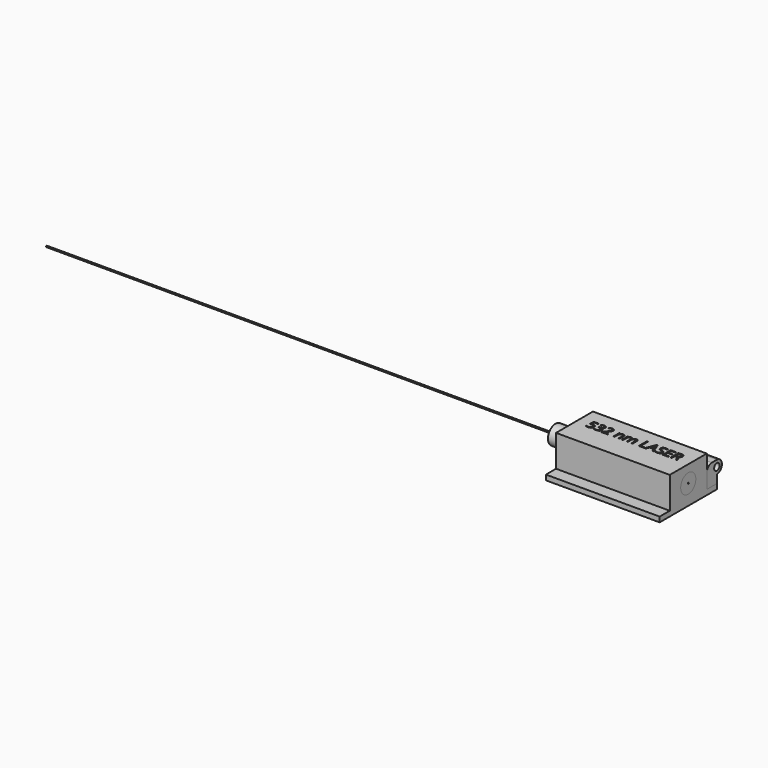
from build123d import *

# Parameters (mm, degrees)
F0_W      = 114.3
F0_H      = 12.7
F1_DEPTH  = 3.81
F3_DEPTH  = 4.572
F4_W      = 114.3
F4_H      = 6.35
F5_DEPTH  = 1.016
F7_DEPTH  = 11.684
F8_R      = 6.34999
F9_R      = 3.429
F9_R_2    = 9.525
F10_DEPTH = 114.301
F2_R      = 3.0988
F11_DEPTH = 10.668
F12_DEPTH = 114.3
F9_R_3    = 0.635
F13_DEPTH = 19.05
F15_DEPTH = 3.175
F16_DEPTH = 114.3
F17_DEPTH = 530.352


# Not quite as in the source:
# - a fillet or chamfer is up to 0.001 mm smaller than in the source, because OpenCascade refuses the exact size


with BuildPart() as f1:
    # F0 (on Top) → F1 (new body)
    with BuildSketch(Plane.XY):
        Rectangle(F0_W, F0_H)
    extrude(amount=F1_DEPTH)

    # F2 (on face) → F3 (join)
    with BuildSketch(Plane.XY.offset(3.81)):
        Polygon((-40.64, 6.2992), (-35.1847327765, 3.1496), (-35.1847327765, -3.1496), (-35.1847327765, -6.35), (35.1847327765, -6.35), (35.1847327765, -3.1496), (35.1847327765, 3.1496), (40.64, 6.2992), (46.0952672235, 3.1496), (46.0952672235, -3.1496), (46.0952672235, -6.35), (57.15, -6.35), (57.15, 6.35), (-57.15, 6.35), (-57.15, -6.35), (-46.0952672235, -6.35), (-46.0952672235, -3.1496), (-46.0952672235, 3.1496), align=None)
    extrude(amount=F3_DEPTH)

    # F4 (on face) → F5 (join)
    with BuildSketch(Plane.XY.offset(8.382)):
        with Locations((0, 9.525)):
            Rectangle(F4_W, F4_H)
        Polygon((-57.15, 6.35), (-57.15, -6.35), (-46.0952672235, -6.35), (-46.0952672235, 3.1496), (-40.64, 6.2992), (-35.1847327765, 3.1496), (-35.1847327765, -6.35), (35.1847327765, -6.35), (35.1847327765, 3.1496), (40.64, 6.2992), (46.0952672235, 3.1496), (46.0952672235, -6.35), (57.15, -6.35), (57.15, 6.35), align=None)
    extrude(amount=F5_DEPTH)

    # F6 (on face) → F7 (join)
    with BuildSketch(Plane.XY.offset(9.398)):
        Polygon((57.15, 12.7), (-57.15, 12.7), (-57.15, -6.35), (-46.0952672235, -6.35), (-46.0952672235, 3.1496), (-40.64, 6.2992), (-35.1847327765, 3.1496), (-35.1847327765, -6.35), (35.1847327765, -6.35), (35.1847327765, 3.1496), (40.64, 6.2992), (46.0952672235, 3.1496), (46.0952672235, -6.35), (57.15, -6.35), align=None)
        Polygon((35.1847327765, -6.35), (46.0952672235, -6.35), (46.0952672235, 3.1496), (40.64, 6.2992), (35.1847327765, 3.1496), align=None)
        Polygon((-46.0952672235, 3.1496), (-46.0952672235, -6.35), (-35.1847327765, -6.35), (-35.1847327765, 3.1496), (-40.64, 6.2992), align=None)
    extrude(amount=F7_DEPTH)

    # F8 (radius 6.35 in the source; OpenCascade refuses exactly that, so slightly less here)
    f8_edges = [f1.edges().sort_by_distance(p)[0] for p in [
        (0, 12.7, 21.082),
        (0, -6.35, 21.082),
        (0, 12.7, 8.382),
    ]]
    fillet(f8_edges, radius=F8_R)

    # F9 (on face) → F10 (cut, through all)
    with BuildSketch(Plane(origin=(-57.15, 0, 0), x_dir=(0, -1, 0), z_dir=(-1, 0, 0))):
        with Locations((-6.35, 14.732)):
            Circle(F9_R)
        Polygon((6.35, 0), (-6.35, 0), (-6.35, -5.1199872978), (65.491868, -5.1199872978), (65.491868, 0), (52.791868, 0), (52.791868, 31.7232050002), (6.35, 31.7232050002), align=None)
        with Locations((29.570934, 14.732)):
            Circle(F9_R_2, mode=Mode.SUBTRACT)
    extrude(amount=-F10_DEPTH, mode=Mode.SUBTRACT)

    # F2 (on face) → F11 (cut, symmetric)
    with BuildSketch(Plane.XY.offset(3.81)):
        with Locations((-40.64, 0)):
            Circle(F2_R)
        with Locations((40.64, 0)):
            Circle(F2_R)
    extrude(amount=F11_DEPTH, both=True, mode=Mode.SUBTRACT)


with BuildPart() as f12:
    # F9 (on face) → F12 (new body)
    with BuildSketch(Plane(origin=(-57.15, 0, 0), x_dir=(0, -1, 0), z_dir=(-1, 0, 0))):
        Polygon((6.35, 0), (-6.35, 0), (-6.35, -5.1199872978), (65.491868, -5.1199872978), (65.491868, 0), (52.791868, 0), (52.791868, 31.7232050002), (6.35, 31.7232050002), (6.35, 14.73201), align=None)
        with Locations((29.570934, 14.732)):
            Circle(F9_R_2, mode=Mode.SUBTRACT)
    extrude(amount=-F12_DEPTH)

    # F9 (on face) → F13 (join, symmetric)
    with BuildSketch(Plane(origin=(-57.15, 0, 0), x_dir=(0, -1, 0), z_dir=(-1, 0, 0))):
        with Locations((29.570934, 14.732)):
            Circle(F9_R_2)
        with Locations((29.570934, 14.732)):
            Circle(F9_R_3, mode=Mode.SUBTRACT)
    extrude(amount=F13_DEPTH, both=True)

    # F14 (on face) → F15 (cut)
    with BuildSketch(Plane.XY.offset(31.7232050002)):
        with BuildLine():
            Line((-45.282163951, -29.570934), (-42.5031012768, -29.570934))
            add(Edge.make_bspline(
                [(-41.0225434028, -28.8201787917), (-41.624680638, -29.3583014371), (-42.5031012768, -29.570934)],
                knots=[0, 0, 0, 0.6048622658, 0.6048622658, 0.6048622658], degree=2))
            add(Edge.make_bspline(
                [(-40.0270486111, -26.3672708056), (-40.0270486111, -27.9305173333), (-41.0225434028, -28.8201787917)],
                knots=[0, 0, 0, 1, 1, 1], degree=2))
            add(Edge.make_bspline(
                [(-40.9398611111, -24.2065069167), (-40.0270486111, -24.9958471944), (-40.0270486111, -26.3672708056)],
                knots=[0, 0, 0, 1, 1, 1], degree=2))
            add(Edge.make_bspline(
                [(-43.4445833333, -23.4171666389), (-41.8526736111, -23.4171666389), (-40.9398611111, -24.2065069167)],
                knots=[0, 0, 0, 1, 1, 1], degree=2))
            add(Edge.make_bspline(
                [(-45.0232638889, -23.5759166389), (-44.23171875, -23.4171666389), (-43.4445833333, -23.4171666389)],
                knots=[0, 0, 0, 1, 1, 1], degree=2))
            Line((-45.0232638889, -23.5759166389), (-44.7675, -20.5508471944))
            Line((-44.7675, -20.5508471944), (-40.7370138889, -20.5508471944))
            Line((-40.7370138889, -20.5508471944), (-40.7370138889, -19.4969235833))
            Line((-40.7370138889, -19.4969235833), (-45.7464583333, -19.4969235833))
            Line((-45.7464583333, -19.4969235833), (-46.1256944444, -24.2109166389))
            Line((-46.1256944444, -24.2109166389), (-45.5325868056, -24.59015275))
            add(Edge.make_bspline(
                [(-43.7819270833, -24.3895103889), (-44.4367708333, -24.3895103889), (-45.5325868056, -24.59015275)],
                knots=[0, 0, 0, 1, 1, 1], degree=2))
            add(Edge.make_bspline(
                [(-41.2000347222, -26.4973576111), (-41.2000347222, -24.3895103889), (-43.7819270833, -24.3895103889)],
                knots=[0, 0, 0, 1, 1, 1], degree=2))
            add(Edge.make_bspline(
                [(-41.8714149306, -28.152105875), (-41.2000347222, -27.5799444167), (-41.2000347222, -26.4973576111)],
                knots=[0, 0, 0, 1, 1, 1], degree=2))
            add(Edge.make_bspline(
                [(-43.75546875, -28.7242673333), (-42.5427951389, -28.7242673333), (-41.8714149306, -28.152105875)],
                knots=[0, 0, 0, 1, 1, 1], degree=2))
            add(Edge.make_bspline(
                [(-45.1687847222, -28.5478784444), (-44.4522048611, -28.7242673333), (-43.75546875, -28.7242673333)],
                knots=[0, 0, 0, 1, 1, 1], degree=2))
            add(Edge.make_bspline(
                [(-46.3660243056, -28.062809), (-45.8853645833, -28.3714895556), (-45.1687847222, -28.5478784444)],
                knots=[0, 0, 0, 1, 1, 1], degree=2))
            Line((-46.3660243056, -28.062809), (-46.3660243056, -29.1652395556))
            add(Edge.make_bspline(
                [(-45.282163951, -29.570934), (-45.9229450337, -29.4347976347), (-46.3660243056, -29.1652395556)],
                knots=[0.5050353738, 0.5050353738, 0.5050353738, 1, 1, 1], degree=2))
        make_face()
        with BuildLine():
            Line((-37.3682522224, -29.570934), (-34.4058239367, -29.570934))
            add(Edge.make_bspline(
                [(-32.9736979167, -28.9337291389), (-33.549949731, -29.3815009681), (-34.4058239367, -29.570934)],
                knots=[0, 0, 0, 0.5769429439, 0.5769429439, 0.5769429439], degree=2))
            add(Edge.make_bspline(
                [(-31.9748958333, -26.7178437222), (-31.9748958333, -28.1576180278), (-32.9736979167, -28.9337291389)],
                knots=[0, 0, 0, 1, 1, 1], degree=2))
            add(Edge.make_bspline(
                [(-32.5602864583, -25.0917586528), (-31.9748958333, -25.7124270556), (-31.9748958333, -26.7178437222)],
                knots=[0, 0, 0, 1, 1, 1], degree=2))
            add(Edge.make_bspline(
                [(-34.3583506944, -24.3211596944), (-33.1456770833, -24.47109025), (-32.5602864583, -25.0917586528)],
                knots=[0, 0, 0, 1, 1, 1], degree=2))
            Line((-34.3583506944, -24.3211596944), (-34.3583506944, -24.2660381667))
            add(Edge.make_bspline(
                [(-32.8248697917, -23.4458298333), (-33.3661631944, -24.0587812222), (-34.3583506944, -24.2660381667)],
                knots=[0, 0, 0, 1, 1, 1], degree=2))
            add(Edge.make_bspline(
                [(-32.2835763889, -21.8671492778), (-32.2835763889, -22.8328784444), (-32.8248697917, -23.4458298333)],
                knots=[0, 0, 0, 1, 1, 1], degree=2))
            add(Edge.make_bspline(
                [(-33.0971701389, -20.0249878194), (-32.2835763889, -20.6963680278), (-32.2835763889, -21.8671492778)],
                knots=[0, 0, 0, 1, 1, 1], degree=2))
            add(Edge.make_bspline(
                [(-35.3769965278, -19.3536076111), (-33.9107638889, -19.3536076111), (-33.0971701389, -20.0249878194)],
                knots=[0, 0, 0, 1, 1, 1], degree=2))
            add(Edge.make_bspline(
                [(-37.0835590278, -19.6325225417), (-36.274375, -19.3536076111), (-35.3769965278, -19.3536076111)],
                knots=[0, 0, 0, 1, 1, 1], degree=2))
            add(Edge.make_bspline(
                [(-38.5123090278, -20.4009166389), (-37.8927430556, -19.9114374722), (-37.0835590278, -19.6325225417)],
                knots=[0, 0, 0, 1, 1, 1], degree=2))
            Line((-38.5123090278, -20.4009166389), (-37.9346354167, -21.1726180278))
            add(Edge.make_bspline(
                [(-36.5973871528, -20.5100572639), (-37.1827777778, -20.6897534444), (-37.9346354167, -21.1726180278)],
                knots=[0, 0, 0, 1, 1, 1], degree=2))
            add(Edge.make_bspline(
                [(-35.3505381944, -20.3303610833), (-36.0119965278, -20.3303610833), (-36.5973871528, -20.5100572639)],
                knots=[0, 0, 0, 1, 1, 1], degree=2))
            add(Edge.make_bspline(
                [(-33.9758072917, -20.7514895556), (-34.4818229167, -20.3303610833), (-35.3505381944, -20.3303610833)],
                knots=[0, 0, 0, 1, 1, 1], degree=2))
            add(Edge.make_bspline(
                [(-33.4697916667, -21.9090416389), (-33.4697916667, -21.1726180278), (-33.9758072917, -20.7514895556)],
                knots=[0, 0, 0, 1, 1, 1], degree=2))
            add(Edge.make_bspline(
                [(-34.1588107639, -23.3532256667), (-33.4697916667, -22.8328784444), (-33.4697916667, -21.9090416389)],
                knots=[0, 0, 0, 1, 1, 1], degree=2))
            add(Edge.make_bspline(
                [(-36.0252256944, -23.8735728889), (-34.8478298611, -23.8735728889), (-34.1588107639, -23.3532256667)],
                knots=[0, 0, 0, 1, 1, 1], degree=2))
            Line((-36.0252256944, -23.8735728889), (-37.0306423611, -23.8735728889))
            Line((-37.0306423611, -23.8735728889), (-37.0306423611, -24.8569409444))
            Line((-37.0306423611, -24.8569409444), (-36.0384548611, -24.8569409444))
            add(Edge.make_bspline(
                [(-33.15890625, -26.6913853889), (-33.15890625, -24.8569409444), (-36.0384548611, -24.8569409444)],
                knots=[0, 0, 0, 1, 1, 1], degree=2))
            add(Edge.make_bspline(
                [(-35.7694618056, -28.7374965), (-33.15890625, -28.7374965), (-33.15890625, -26.6913853889)],
                knots=[0, 0, 0, 1, 1, 1], degree=2))
            add(Edge.make_bspline(
                [(-37.1717534722, -28.568824625), (-36.4309201389, -28.7374965), (-35.7694618056, -28.7374965)],
                knots=[0, 0, 0, 1, 1, 1], degree=2))
            add(Edge.make_bspline(
                [(-38.5674305556, -28.0760381667), (-37.9125868056, -28.40015275), (-37.1717534722, -28.568824625)],
                knots=[0, 0, 0, 1, 1, 1], degree=2))
            Line((-38.5674305556, -28.0760381667), (-38.5674305556, -29.1652395556))
            add(Edge.make_bspline(
                [(-37.3682522224, -29.570934), (-37.9845576037, -29.4464141838), (-38.5674305556, -29.1652395556)],
                knots=[0.0691615274, 0.0691615274, 0.0691615274, 1, 1, 1], degree=2))
        make_face()
        with BuildLine():
            Line((-30.4579513889, -28.5853610833), (-30.4579513889, -29.570934))
            Line((-30.4579513889, -29.570934), (-23.8367534722, -29.570934))
            Line((-23.8367534722, -29.570934), (-23.8367534722, -28.5103958056))
            Line((-23.8367534722, -28.5103958056), (-29.0181770833, -28.5103958056))
            Line((-29.0181770833, -28.5103958056), (-29.0181770833, -28.4552742778))
            Line((-29.0181770833, -28.4552742778), (-26.8133159722, -26.2989201111))
            add(Edge.make_bspline(
                [(-24.8024826389, -23.9286944167), (-25.34046875, -24.8657603889), (-26.8133159722, -26.2989201111)],
                knots=[0, 0, 0, 1, 1, 1], degree=2))
            add(Edge.make_bspline(
                [(-24.2644965278, -22.0325138611), (-24.2644965278, -22.9916284444), (-24.8024826389, -23.9286944167)],
                knots=[0, 0, 0, 1, 1, 1], degree=2))
            add(Edge.make_bspline(
                [(-25.0703732639, -20.0801093472), (-24.2644965278, -20.8066110833), (-24.2644965278, -22.0325138611)],
                knots=[0, 0, 0, 1, 1, 1], degree=2))
            add(Edge.make_bspline(
                [(-27.2961805556, -19.3536076111), (-25.87625, -19.3536076111), (-25.0703732639, -20.0801093472)],
                knots=[0, 0, 0, 1, 1, 1], degree=2))
            add(Edge.make_bspline(
                [(-30.3278645833, -20.5111596944), (-28.9365972222, -19.3536076111), (-27.2961805556, -19.3536076111)],
                knots=[0, 0, 0, 1, 1, 1], degree=2))
            Line((-30.3278645833, -20.5111596944), (-29.7215277778, -21.2894756667))
            add(Edge.make_bspline(
                [(-28.4713715278, -20.5376180278), (-29.0336111111, -20.7448749722), (-29.7215277778, -21.2894756667)],
                knots=[0, 0, 0, 1, 1, 1], degree=2))
            add(Edge.make_bspline(
                [(-27.2829513889, -20.3303610833), (-27.9091319444, -20.3303610833), (-28.4713715278, -20.5376180278)],
                knots=[0, 0, 0, 1, 1, 1], degree=2))
            add(Edge.make_bspline(
                [(-25.9247569444, -20.8022013611), (-26.4142361111, -20.3303610833), (-27.2829513889, -20.3303610833)],
                knots=[0, 0, 0, 1, 1, 1], degree=2))
            add(Edge.make_bspline(
                [(-25.4352777778, -22.0810208056), (-25.4352777778, -21.2740416389), (-25.9247569444, -20.8022013611)],
                knots=[0, 0, 0, 1, 1, 1], degree=2))
            add(Edge.make_bspline(
                [(-25.628203125, -23.1481735833), (-25.4352777778, -22.6520798333), (-25.4352777778, -22.0810208056)],
                knots=[0, 0, 0, 1, 1, 1], degree=2))
            add(Edge.make_bspline(
                [(-26.2069791667, -24.1679218472), (-25.8211284722, -23.6442673333), (-25.628203125, -23.1481735833)],
                knots=[0, 0, 0, 1, 1, 1], degree=2))
            add(Edge.make_bspline(
                [(-27.8055034722, -25.919684), (-26.5928298611, -24.6915763611), (-26.2069791667, -24.1679218472)],
                knots=[0, 0, 0, 1, 1, 1], degree=2))
            Line((-27.8055034722, -25.919684), (-30.4579513889, -28.5853610833))
        make_face()
        with BuildLine():
            Line((-18.2011284722, -22.0192846944), (-18.2011284722, -29.570934))
            Line((-18.2011284722, -29.570934), (-17.0568055556, -29.570934))
            Line((-17.0568055556, -29.570934), (-17.0568055556, -25.6087985833))
            add(Edge.make_bspline(
                [(-16.5055902778, -23.4932343472), (-17.0568055556, -24.1337465), (-17.0568055556, -25.6087985833)],
                knots=[0, 0, 0, 1, 1, 1], degree=2))
            add(Edge.make_bspline(
                [(-14.7703645833, -22.8527221944), (-15.954375, -22.8527221944), (-16.5055902778, -23.4932343472)],
                knots=[0, 0, 0, 1, 1, 1], degree=2))
            add(Edge.make_bspline(
                [(-13.4529600694, -23.3080260139), (-13.8729861111, -22.8527221944), (-14.7703645833, -22.8527221944)],
                knots=[0, 0, 0, 1, 1, 1], degree=2))
            add(Edge.make_bspline(
                [(-13.0329340278, -24.6849617778), (-13.0329340278, -23.7633298333), (-13.4529600694, -23.3080260139)],
                knots=[0, 0, 0, 1, 1, 1], degree=2))
            Line((-13.0329340278, -24.6849617778), (-13.0329340278, -29.570934))
            Line((-13.0329340278, -29.570934), (-11.8886111111, -29.570934))
            Line((-11.8886111111, -29.570934), (-11.8886111111, -24.6452742778))
            add(Edge.make_bspline(
                [(-12.5776302083, -22.5385294861), (-11.8886111111, -23.1966805278), (-11.8886111111, -24.6452742778)],
                knots=[0, 0, 0, 1, 1, 1], degree=2))
            add(Edge.make_bspline(
                [(-14.6314583333, -21.8803784444), (-13.2666493056, -21.8803784444), (-12.5776302083, -22.5385294861)],
                knots=[0, 0, 0, 1, 1, 1], degree=2))
            add(Edge.make_bspline(
                [(-16.043671875, -22.1879565694), (-15.4097743056, -21.8803784444), (-14.6314583333, -21.8803784444)],
                knots=[0, 0, 0, 1, 1, 1], degree=2))
            add(Edge.make_bspline(
                [(-17.0303472222, -23.0533645556), (-16.6775694444, -22.4955346944), (-16.043671875, -22.1879565694)],
                knots=[0, 0, 0, 1, 1, 1], degree=2))
            Line((-17.0303472222, -23.0533645556), (-17.08546875, -23.0533645556))
            Line((-17.08546875, -23.0533645556), (-17.2706770833, -22.0192846944))
            Line((-17.2706770833, -22.0192846944), (-18.2011284722, -22.0192846944))
        make_face()
        with BuildLine():
            Line((-9.5404340278, -22.0192846944), (-9.5404340278, -29.570934))
            Line((-9.5404340278, -29.570934), (-8.3961111111, -29.570934))
            Line((-8.3961111111, -29.570934), (-8.3961111111, -25.6087985833))
            add(Edge.make_bspline(
                [(-7.8967100694, -23.4965416389), (-8.3961111111, -24.1403610833), (-8.3961111111, -25.6087985833)],
                knots=[0, 0, 0, 1, 1, 1], degree=2))
            add(Edge.make_bspline(
                [(-6.3235416667, -22.8527221944), (-7.3973090278, -22.8527221944), (-7.8967100694, -23.4965416389)],
                knots=[0, 0, 0, 1, 1, 1], degree=2))
            add(Edge.make_bspline(
                [(-5.1174826389, -23.3036162917), (-5.5033333333, -22.8527221944), (-6.3235416667, -22.8527221944)],
                knots=[0, 0, 0, 1, 1, 1], degree=2))
            add(Edge.make_bspline(
                [(-4.7316319444, -24.6585034444), (-4.7316319444, -23.7545103889), (-5.1174826389, -23.3036162917)],
                knots=[0, 0, 0, 1, 1, 1], degree=2))
            Line((-4.7316319444, -24.6585034444), (-4.7316319444, -29.570934))
            Line((-4.7316319444, -29.570934), (-3.5873090278, -29.570934))
            Line((-3.5873090278, -29.570934), (-3.5873090278, -25.3530346944))
            add(Edge.make_bspline(
                [(-3.0768836806, -23.4656735833), (-3.5873090278, -24.0786249722), (-3.5873090278, -25.3530346944)],
                knots=[0, 0, 0, 1, 1, 1], degree=2))
            add(Edge.make_bspline(
                [(-1.4993055556, -22.8527221944), (-2.5664583333, -22.8527221944), (-3.0768836806, -23.4656735833)],
                knots=[0, 0, 0, 1, 1, 1], degree=2))
            add(Edge.make_bspline(
                [(-0.2998611111, -23.3036162917), (-0.6857118056, -22.8527221944), (-1.4993055556, -22.8527221944)],
                knots=[0, 0, 0, 1, 1, 1], degree=2))
            add(Edge.make_bspline(
                [(0.0859895833, -24.6585034444), (0.0859895833, -23.7545103889), (-0.2998611111, -23.3036162917)],
                knots=[0, 0, 0, 1, 1, 1], degree=2))
            Line((0.0859895833, -24.6585034444), (0.0859895833, -29.570934))
            Line((0.0859895833, -29.570934), (1.2281076389, -29.570934))
            Line((1.2281076389, -29.570934), (1.2281076389, -24.6452742778))
            add(Edge.make_bspline(
                [(0.5909027778, -22.5385294861), (1.2281076389, -23.1966805278), (1.2281076389, -24.6452742778)],
                knots=[0, 0, 0, 1, 1, 1], degree=2))
            add(Edge.make_bspline(
                [(-1.3273263889, -21.8803784444), (-0.0463020833, -21.8803784444), (0.5909027778, -22.5385294861)],
                knots=[0, 0, 0, 1, 1, 1], degree=2))
            add(Edge.make_bspline(
                [(-2.788046875, -22.2254392083), (-2.1475347222, -21.8803784444), (-1.3273263889, -21.8803784444)],
                knots=[0, 0, 0, 1, 1, 1], degree=2))
            add(Edge.make_bspline(
                [(-3.7659027778, -23.1636076111), (-3.4285590278, -22.5704999722), (-2.788046875, -22.2254392083)],
                knots=[0, 0, 0, 1, 1, 1], degree=2))
            Line((-3.7659027778, -23.1636076111), (-3.8210243056, -23.1636076111))
            add(Edge.make_bspline(
                [(-6.1361284722, -21.8803784444), (-4.365625, -21.8803784444), (-3.8210243056, -23.1636076111)],
                knots=[0, 0, 0, 1, 1, 1], degree=2))
            add(Edge.make_bspline(
                [(-7.4557378472, -22.1912638611), (-6.8659375, -21.8803784444), (-6.1361284722, -21.8803784444)],
                knots=[0, 0, 0, 1, 1, 1], degree=2))
            add(Edge.make_bspline(
                [(-8.3696527778, -23.0533645556), (-8.0455381944, -22.5021492778), (-7.4557378472, -22.1912638611)],
                knots=[0, 0, 0, 1, 1, 1], degree=2))
            Line((-8.3696527778, -23.0533645556), (-8.4247743056, -23.0533645556))
            Line((-8.4247743056, -23.0533645556), (-8.6099826389, -22.0192846944))
            Line((-8.6099826389, -22.0192846944), (-9.5404340278, -22.0192846944))
        make_face()
        Polygon((7.4237673611, -19.4969235833), (7.4237673611, -29.570934), (13.0395486111, -29.570934), (13.0395486111, -28.5103958056), (8.5945486111, -28.5103958056), (8.5945486111, -19.4969235833), align=None)
        Polygon((17.3456423611, -19.4550312222), (13.3636631944, -29.570934), (14.5498784722, -29.570934), (15.7890104167, -26.3672708056), (19.8261111111, -26.3672708056), (21.0806770833, -29.570934), (22.2933506944, -29.570934), (18.3312152778, -19.4550312222), align=None)
        with BuildLine():
            Line((18.2893229167, -22.1912638611), (19.4623090278, -25.3133471944))
            Line((19.4623090278, -25.3133471944), (16.2035243056, -25.3133471944))
            Line((16.2035243056, -25.3133471944), (17.3875347222, -22.1912638611))
            add(Edge.make_bspline(
                [(17.8218923611, -20.7382603889), (17.6697569444, -21.3997187222), (17.3875347222, -22.1912638611)],
                knots=[0, 0, 0, 1, 1, 1], degree=2))
            add(Edge.make_bspline(
                [(18.2893229167, -22.1912638611), (18.0622222222, -21.5981562222), (17.8218923611, -20.7382603889)],
                knots=[0, 0, 0, 1, 1, 1], degree=2))
        make_face(mode=Mode.SUBTRACT)
        with BuildLine():
            Line((24.065394409, -29.570934), (27.0786655087, -29.570934))
            add(Edge.make_bspline(
                [(28.3975086806, -28.9645971944), (27.8493399544, -29.3880966903), (27.0786655087, -29.570934)],
                knots=[0, 0, 0, 0.5682703015, 0.5682703015, 0.5682703015], degree=2))
            add(Edge.make_bspline(
                [(29.3621354167, -26.8898228889), (29.3621354167, -28.2193541389), (28.3975086806, -28.9645971944)],
                knots=[0, 0, 0, 1, 1, 1], degree=2))
            add(Edge.make_bspline(
                [(28.7668229167, -25.2097187222), (29.3621354167, -25.8579478889), (29.3621354167, -26.8898228889)],
                knots=[0, 0, 0, 1, 1, 1], degree=2))
            add(Edge.make_bspline(
                [(26.5862152778, -23.9970451111), (28.1715104167, -24.5614895556), (28.7668229167, -25.2097187222)],
                knots=[0, 0, 0, 1, 1, 1], degree=2))
            add(Edge.make_bspline(
                [(25.1839236111, -23.3807864306), (25.6425347222, -23.6597013611), (26.5862152778, -23.9970451111)],
                knots=[0, 0, 0, 1, 1, 1], degree=2))
            add(Edge.make_bspline(
                [(24.5323871528, -22.7667326111), (24.7253125, -23.1018715), (25.1839236111, -23.3807864306)],
                knots=[0, 0, 0, 1, 1, 1], degree=2))
            add(Edge.make_bspline(
                [(24.3394618056, -21.9090416389), (24.3394618056, -22.4315937222), (24.5323871528, -22.7667326111)],
                knots=[0, 0, 0, 1, 1, 1], degree=2))
            add(Edge.make_bspline(
                [(24.8631163194, -20.7999965), (24.3394618056, -21.1990763611), (24.3394618056, -21.9090416389)],
                knots=[0, 0, 0, 1, 1, 1], degree=2))
            add(Edge.make_bspline(
                [(26.3172222222, -20.4009166389), (25.3867708333, -20.4009166389), (24.8631163194, -20.7999965)],
                knots=[0, 0, 0, 1, 1, 1], degree=2))
            add(Edge.make_bspline(
                [(28.7425694444, -20.9234687222), (27.4946180556, -20.4009166389), (26.3172222222, -20.4009166389)],
                knots=[0, 0, 0, 1, 1, 1], degree=2))
            Line((28.7425694444, -20.9234687222), (29.1085763889, -19.9048228889))
            add(Edge.make_bspline(
                [(26.3458854167, -19.3536076111), (27.8473958333, -19.3536076111), (29.1085763889, -19.9048228889)],
                knots=[0, 0, 0, 1, 1, 1], degree=2))
            add(Edge.make_bspline(
                [(24.0296788194, -20.0426267083), (24.90390625, -19.3536076111), (26.3458854167, -19.3536076111)],
                knots=[0, 0, 0, 1, 1, 1], degree=2))
            add(Edge.make_bspline(
                [(23.1554513889, -21.8958124722), (23.1554513889, -20.7316458056), (24.0296788194, -20.0426267083)],
                knots=[0, 0, 0, 1, 1, 1], degree=2))
            add(Edge.make_bspline(
                [(23.7584809028, -23.6938767083), (23.1554513889, -23.0048576111), (23.1554513889, -21.8958124722)],
                knots=[0, 0, 0, 1, 1, 1], degree=2))
            add(Edge.make_bspline(
                [(25.7660069444, -24.8856041389), (24.3615104167, -24.3828958056), (23.7584809028, -23.6938767083)],
                knots=[0, 0, 0, 1, 1, 1], degree=2))
            add(Edge.make_bspline(
                [(27.2642100694, -25.5261162917), (26.7714236111, -25.2427916389), (25.7660069444, -24.8856041389)],
                knots=[0, 0, 0, 1, 1, 1], degree=2))
            add(Edge.make_bspline(
                [(27.9675607639, -26.1434774028), (27.7569965278, -25.8094409444), (27.2642100694, -25.5261162917)],
                knots=[0, 0, 0, 1, 1, 1], degree=2))
            add(Edge.make_bspline(
                [(28.178125, -27.0000659444), (28.178125, -26.4775138611), (27.9675607639, -26.1434774028)],
                knots=[0, 0, 0, 1, 1, 1], degree=2))
            add(Edge.make_bspline(
                [(27.5850173611, -28.2380954583), (28.178125, -27.7938159444), (28.178125, -27.0000659444)],
                knots=[0, 0, 0, 1, 1, 1], degree=2))
            add(Edge.make_bspline(
                [(25.8211284722, -28.6823749722), (26.9919097222, -28.6823749722), (27.5850173611, -28.2380954583)],
                knots=[0, 0, 0, 1, 1, 1], degree=2))
            add(Edge.make_bspline(
                [(24.3747395833, -28.5302395556), (25.1045486111, -28.6823749722), (25.8211284722, -28.6823749722)],
                knots=[0, 0, 0, 1, 1, 1], degree=2))
            add(Edge.make_bspline(
                [(23.0231597222, -28.1179305278), (23.6449305556, -28.3781041389), (24.3747395833, -28.5302395556)],
                knots=[0, 0, 0, 1, 1, 1], degree=2))
            Line((23.0231597222, -28.1179305278), (23.0231597222, -29.2468194167))
            add(Edge.make_bspline(
                [(24.065394409, -29.570934), (23.4599372399, -29.456233295), (23.0231597222, -29.2468194167)],
                knots=[0.5477225575, 0.5477225575, 0.5477225575, 1, 1, 1], degree=2))
        make_face()
        Polygon((31.4236805556, -29.570934), (37.0394618056, -29.570934), (37.0394618056, -28.5236249722), (32.5944618056, -28.5236249722), (32.5944618056, -24.8172534444), (36.77046875, -24.8172534444), (36.77046875, -23.7831735833), (32.5944618056, -23.7831735833), (32.5944618056, -20.5376180278), (37.0394618056, -20.5376180278), (37.0394618056, -19.4969235833), (31.4236805556, -19.4969235833), align=None)
        with BuildLine():
            Line((44.9835763889, -29.570934), (46.3682291667, -29.570934))
            Line((46.3682291667, -29.570934), (43.6319965278, -25.0443541389))
            add(Edge.make_bspline(
                [(45.6582638889, -22.3433992778), (45.6582638889, -24.3410034444), (43.6319965278, -25.0443541389)],
                knots=[0, 0, 0, 1, 1, 1], degree=2))
            add(Edge.make_bspline(
                [(44.7730121528, -20.2068888611), (45.6582638889, -20.9168541389), (45.6582638889, -22.3433992778)],
                knots=[0, 0, 0, 1, 1, 1], degree=2))
            add(Edge.make_bspline(
                [(42.0334722222, -19.4969235833), (43.8877604167, -19.4969235833), (44.7730121528, -20.2068888611)],
                knots=[0, 0, 0, 1, 1, 1], degree=2))
            Line((42.0334722222, -19.4969235833), (39.27078125, -19.4969235833))
            Line((39.27078125, -19.4969235833), (39.27078125, -29.570934))
            Line((39.27078125, -29.570934), (40.4415625, -29.570934))
            Line((40.4415625, -29.570934), (40.4415625, -25.3816978889))
            Line((40.4415625, -25.3816978889), (42.545, -25.3816978889))
            Line((42.545, -25.3816978889), (44.9835763889, -29.570934))
        make_face()
        with BuildLine():
            Line((42.04890625, -24.3762812222), (40.4415625, -24.3762812222))
            Line((40.4415625, -24.3762812222), (40.4415625, -20.5243888611))
            Line((40.4415625, -20.5243888611), (41.9651215278, -20.5243888611))
            add(Edge.make_bspline(
                [(43.8568923611, -20.9653610833), (43.2681944444, -20.5243888611), (41.9651215278, -20.5243888611)],
                knots=[0, 0, 0, 1, 1, 1], degree=2))
            add(Edge.make_bspline(
                [(44.4455902778, -22.4051353889), (44.4455902778, -21.4063333056), (43.8568923611, -20.9653610833)],
                knots=[0, 0, 0, 1, 1, 1], degree=2))
            add(Edge.make_bspline(
                [(43.8668142361, -23.8834947639), (44.4455902778, -23.3907083056), (44.4455902778, -22.4051353889)],
                knots=[0, 0, 0, 1, 1, 1], degree=2))
            add(Edge.make_bspline(
                [(42.04890625, -24.3762812222), (43.2880381944, -24.3762812222), (43.8668142361, -23.8834947639)],
                knots=[0, 0, 0, 1, 1, 1], degree=2))
        make_face(mode=Mode.SUBTRACT)
    extrude(amount=-F15_DEPTH, mode=Mode.SUBTRACT)

    # F9 (on face) → F16 (join)
    with BuildSketch(Plane(origin=(-57.15, 0, 0), x_dir=(0, -1, 0), z_dir=(-1, 0, 0))):
        with Locations((29.570934, 14.732)):
            Circle(F9_R_2)
        with Locations((29.570934, 14.732)):
            Circle(F9_R_3, mode=Mode.SUBTRACT)
    extrude(amount=-F16_DEPTH)


with BuildPart() as f17:
    # F9 (on face) → F17 (new body)
    with BuildSketch(Plane(origin=(-57.15, 0, 0), x_dir=(0, -1, 0), z_dir=(-1, 0, 0))):
        with Locations((29.570934, 14.732)):
            Circle(F9_R_3)
    extrude(amount=F17_DEPTH)


solid = Compound([f1.part, f12.part, f17.part])
